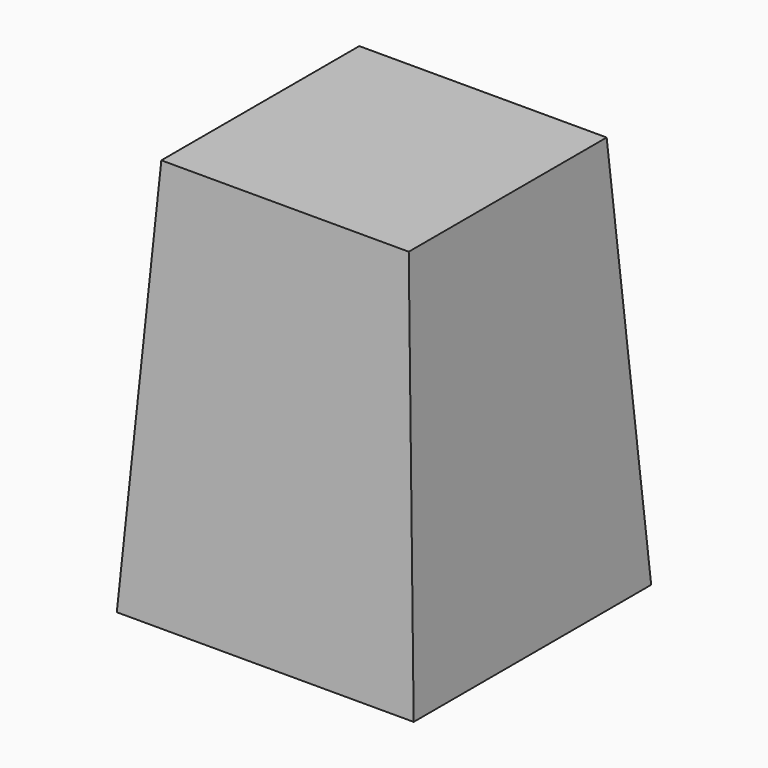
from build123d import *

# Parameters (mm, degrees)
F0_W     = 76.2
F0_H     = 76.2
F1_DEPTH = 101.6
F2_SIZE2 = 101.59999
F2_SIZE  = 6.34999


# Not quite as in the source:
# - a fillet or chamfer is up to 0.001 mm smaller than in the source, because OpenCascade refuses the exact size


with BuildPart() as f1:
    # F0 (on Top) → F1 (new body)
    with BuildSketch(Plane.XY):
        with Locations((-38.1, 38.1)):
            Rectangle(F0_W, F0_H)
    extrude(amount=F1_DEPTH)

    # F2 (size 6.35 and 101.6 in the source; OpenCascade refuses exactly that, so slightly less here)
    f2_edges = [f1.edges().sort_by_distance(p)[0] for p in [
        (-38.1, 0, 101.6),
        (-76.2, 38.1, 101.6),
        (0, 38.1, 101.6),
        (-38.1, 76.2, 101.6),
    ]]
    f2_side = f1.faces().sort_by_distance((-38.1, 38.1, 101.6))[0]
    chamfer(f2_edges, length=F2_SIZE, length2=F2_SIZE2, reference=f2_side)


solid = f1.part
